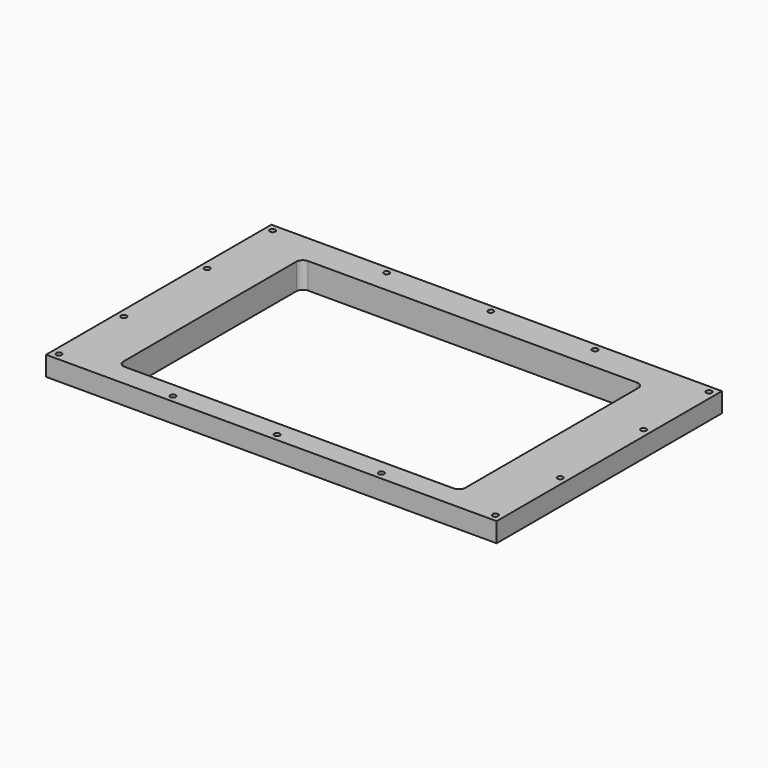
from build123d import *

# Parameters (mm, degrees)
F1_DEPTH = 3.175
F2_W     = 219.71
F2_H     = 137.3124
F3_DEPTH = 9.525
F5_D     = 2.7051


# Not quite as in the source:
# - a feature of the source that left no trace in its solid (it failed there, or was rolled back) is left out


with BuildPart() as f1:
    # F0 (on Top) → F1 (new body)
    with BuildSketch(Plane.XY):
        with BuildLine():
            ThreePointArc((100.71989, 56.515), (98.8600180605, 61.0051280605), (94.36989, 62.865))
            Line((94.36989, 62.865), (-94.36989, 62.865))
            ThreePointArc((-94.36989, 62.865), (-98.8600180605, 61.0051280605), (-100.71989, 56.515))
            Line((-100.71989, 56.515), (-100.71989, -56.515))
            ThreePointArc((-100.71989, -56.515), (-98.8600180605, -61.0051280605), (-94.36989, -62.865))
            Line((-94.36989, -62.865), (94.36989, -62.865))
            ThreePointArc((94.36989, -62.865), (98.8600180605, -61.0051280605), (100.71989, -56.515))
            Line((100.71989, -56.515), (100.71989, 56.515))
        make_face()
        with BuildLine():
            ThreePointArc((83.3755, -54.61), (82.4455640303, -56.8550640303), (80.2005, -57.785))
            Line((80.2005, -57.785), (-80.2005, -57.785))
            ThreePointArc((-80.2005, -57.785), (-82.4455640303, -56.8550640303), (-83.3755, -54.61))
            Line((-83.3755, -54.61), (-83.3755, 50.8))
            ThreePointArc((-83.3755, 50.8), (-82.4455640303, 53.0450640303), (-80.2005, 53.975))
            Line((-80.2005, 53.975), (80.2005, 53.975))
            ThreePointArc((80.2005, 53.975), (82.4455640303, 53.0450640303), (83.3755, 50.8))
            Line((83.3755, 50.8), (83.3755, -54.61))
        make_face(mode=Mode.SUBTRACT)
    extrude(amount=-F1_DEPTH)

    # F2 (on face) → F3 (join)
    with BuildSketch(Plane.XY):
        Rectangle(F2_W, F2_H)
        with BuildLine():
            Line((-80.2005, 53.975), (80.2005, 53.975))
            ThreePointArc((80.2005, 53.975), (82.4455640303, 53.0450640303), (83.3755, 50.8))
            Line((83.3755, 50.8), (83.3755, -54.61))
            ThreePointArc((83.3755, -54.61), (82.4455640303, -56.8550640303), (80.2005, -57.785))
            Line((80.2005, -57.785), (-80.2005, -57.785))
            ThreePointArc((-80.2005, -57.785), (-82.4455640303, -56.8550640303), (-83.3755, -54.61))
            Line((-83.3755, -54.61), (-83.3755, 50.8))
            ThreePointArc((-83.3755, 50.8), (-82.4455640303, 53.0450640303), (-80.2005, 53.975))
        make_face(mode=Mode.SUBTRACT)
    extrude(amount=F3_DEPTH)

    # F5 (through all)
    with Locations(Plane(origin=(0, 0, 0), x_dir=(1, 0, 0), z_dir=(0, 0, -1))):
        with Locations((106.4006, -65.1256), (50.8, -65.1256), (0, -65.1256), (-50.8, -65.1256), (-106.4006, -65.1256), (-106.4006, -25.2095), (-106.4006, 25.5905), (-106.4006, 65.1256), (0, 65.1256), (-50.8, 65.1256), (50.8, 65.1256), (106.4006, 65.1256), (106.4006, 25.5905), (106.4006, -25.2095)):
            Hole(F5_D / 2)


solid = f1.part
